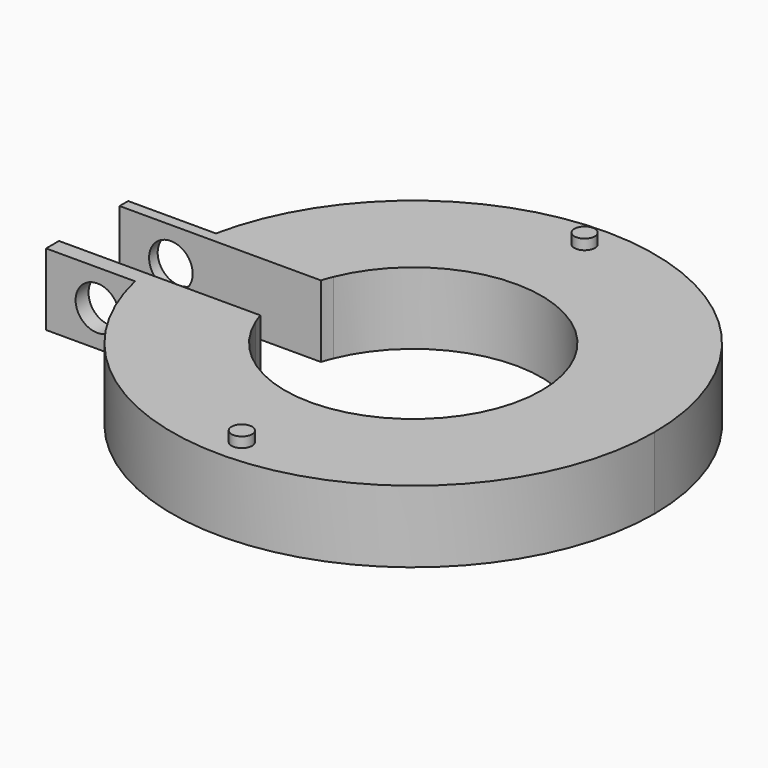
from build123d import *

# Parameters (mm, degrees)
F1_DEPTH = 7
F2_R     = 2.125
F3_DEPTH = 10
F4_R     = 1
F5_DEPTH = 1


# Not quite as in the source:
# - a feature names something its author has since deleted; it is built from what else it names


with BuildPart() as f1:
    # F0 (on Top) → F1 (new body)
    with BuildSketch(Plane.XY):
        with BuildLine():
            ThreePointArc((-23.208916684, 3.6873006871), (-23.1191027664, 4.2139159074), (-23.017341427, 4.7383534726))
            Line((-23.017341427, 4.7383534726), (-31.5671088163, 4.7383534726))
            Line((-31.5671088163, 4.7383534726), (-31.5671088163, 3.6873006871))
            Line((-31.5671088163, 3.6873006871), (-23.208916684, 3.6873006871))
        make_face()
        with BuildLine():
            Line((-31.5671088163, -5.2616465274), (-22.9033856847, -5.2616465274))
            ThreePointArc((-22.9033856847, -5.2616465274), (-23.0695849256, -4.4770806738), (-23.208916684, -3.6873006871))
            Line((-23.208916684, -3.6873006871), (-31.5671088163, -3.6873006871))
            Line((-31.5671088163, -3.6873006871), (-31.5671088163, -5.2616465274))
        make_face()
        with BuildLine():
            ThreePointArc((-22.9033856847, -5.2616465274), (2.6476816661, -23.3503700569), (23.5, 0))
            ThreePointArc((23.5, 0), (2.3814361701, 23.3790239695), (-23.017341427, 4.7383534726))
            Line((-23.017341427, 4.7383534726), (-11.5671088163, 4.7383534726))
            ThreePointArc((-11.5671088163, 4.7383534726), (2.4146573045, 12.2645599229), (12.5, 0))
            ThreePointArc((12.5, 0), (2.4146573045, -12.2645599229), (-11.5671088163, -4.7383534726))
            Line((-11.5671088163, -4.7383534726), (-11.5671088163, -5.2616465274))
            Line((-11.5671088163, -5.2616465274), (-22.9033856847, -5.2616465274))
        make_face()
        with BuildLine():
            Line((-11.5671088163, 4.7383534726), (-23.017341427, 4.7383534726))
            ThreePointArc((-23.017341427, 4.7383534726), (-23.1191027664, 4.2139159074), (-23.208916684, 3.6873006871))
            Line((-23.208916684, 3.6873006871), (-11.9437771933, 3.6873006871))
            ThreePointArc((-11.9437771933, 3.6873006871), (-11.7671839549, 4.2170347131), (-11.5671088163, 4.7383534726))
        make_face()
        with BuildLine():
            ThreePointArc((-23.208916684, -3.6873006871), (-23.0695849256, -4.4770806738), (-22.9033856847, -5.2616465274))
            Line((-22.9033856847, -5.2616465274), (-11.5671088163, -5.2616465274))
            Line((-11.5671088163, -5.2616465274), (-11.5671088163, -4.7383534726))
            ThreePointArc((-11.5671088163, -4.7383534726), (-11.7671839549, -4.2170347131), (-11.9437771933, -3.6873006871))
            Line((-11.9437771933, -3.6873006871), (-23.208916684, -3.6873006871))
        make_face()
    extrude(amount=F1_DEPTH)

    # F2 (on face) → F3 (cut)
    with BuildSketch(Plane.XZ.offset(5.2616465274)):
        with Locations((-26.5671088163, 3.5)):
            Circle(F2_R)
    extrude(amount=-F3_DEPTH, mode=Mode.SUBTRACT)

    # F4 (on face) → F5 (join, symmetric)
    with BuildSketch(Plane.XY.offset(7)):
        with Locations((0, -20.875)):
            Circle(F4_R)
        with Locations((0, 20.875)):
            Circle(F4_R)
    extrude(amount=F5_DEPTH, both=True)


solid = f1.part
